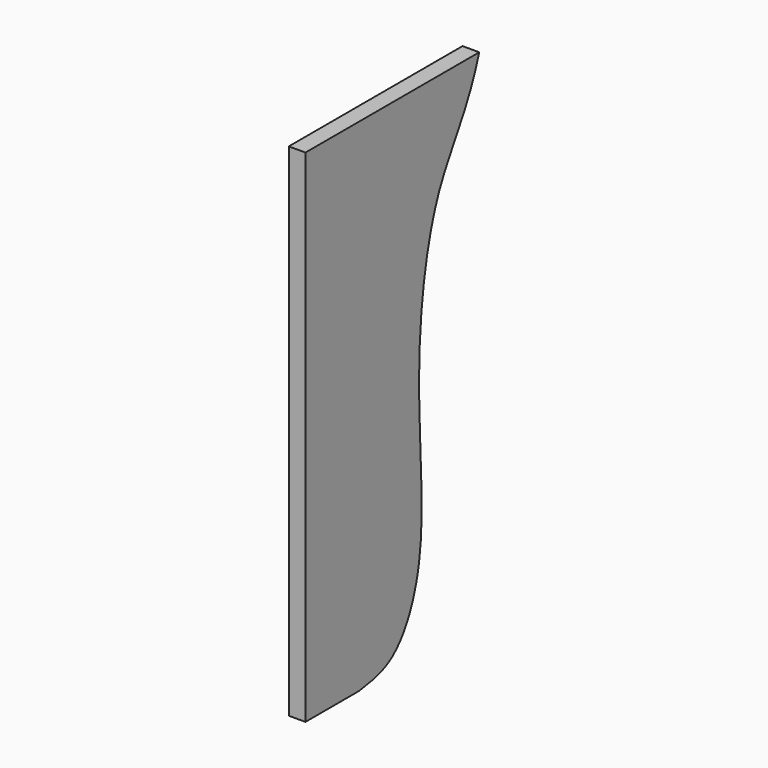
from build123d import *

# Parameters (mm, degrees)
F0_W     = 82.55
F0_H     = 190.5
F1_DEPTH = 6.35
F2_W     = 22.225
F2_H     = 5.08
F2_W_2   = 19.05
F2_H_2   = 26.4446459055
F2_H_3   = 61.5272244272
F2_H_4   = 58.6440721527
F3_DEPTH = 12.7


# Not quite as in the source:
# - a feature names something its author has since deleted; it is built from what else it names


with BuildPart() as f1:
    # F0 (on Right) → F1 (new body)
    with BuildSketch(Plane.YZ):
        with Locations((-52.8816960618, -14.7416193426)):
            Rectangle(F0_W, F0_H)
    extrude(amount=F1_DEPTH)

    # F2 (on face) → F3 (cut)
    with BuildSketch(Plane.YZ.offset(6.35)):
        with BuildLine():
            add(Edge.make_bspline(
                [(-52.8816960618, -104.9116193426), (-46.7384052574, -100.1821825443), (-42.1059434018, -90.4449211167), (-40.1816960618, -78.4669734371)],
                knots=[0.1290930094, 0.1290930094, 0.1290930094, 0.1290930094, 0.3003556222, 0.3003556222, 0.3003556222, 0.3003556222], degree=3))
            Line((-52.8816960618, -104.9116193426), (-30.6566960618, -104.9116193426))
            Line((-30.6566960618, -104.9116193426), (-30.6566960618, -78.4669734371))
            Line((-30.6566960618, -78.4669734371), (-40.1816960618, -78.4669734371))
        make_face()
        with Locations((-41.7691960618, -107.4516193426)):
            Rectangle(F2_W, F2_H)
        with BuildLine():
            add(Edge.make_bspline(
                [(-68.7566960618, -109.9916193426), (-63.0013923205, -109.1961470607), (-57.5123383521, -108.4765376811), (-52.8816960618, -104.9116193426)],
                knots=[0, 0, 0, 0, 0.1290930094, 0.1290930094, 0.1290930094, 0.1290930094], degree=3))
            Line((-68.7566960618, -109.9916193426), (-52.8816960618, -109.9916193426))
            Line((-52.8816960618, -109.9916193426), (-52.8816960618, -104.9116193426))
        make_face()
        with Locations((-21.1316960618, -107.4516193426)):
            Rectangle(F2_W_2, F2_H)
        with Locations((-21.1316960618, -91.6892963898)):
            Rectangle(F2_W_2, F2_H_2)
        with Locations((-21.1316960618, -47.7033612235)):
            Rectangle(F2_W_2, F2_H_3)
        with BuildLine():
            add(Edge.make_bspline(
                [(-40.1816960618, -78.4669734371), (-37.3949778969, -61.1203653983), (-40.2882470853, -39.0743255012), (-40.1816960618, -16.9397490099)],
                knots=[0.3003556222, 0.3003556222, 0.3003556222, 0.3003556222, 0.5483802, 0.5483802, 0.5483802, 0.5483802], degree=3))
            Line((-40.1816960618, -78.4669734371), (-30.6566960618, -78.4669734371))
            Line((-30.6566960618, -78.4669734371), (-30.6566960618, -16.9397490099))
            Line((-30.6566960618, -16.9397490099), (-40.1816960618, -16.9397490099))
        make_face()
        with BuildLine():
            add(Edge.make_bspline(
                [(-40.1816960618, -16.9397490099), (-40.0769921004, 4.8111245801), (-37.0755702459, 26.6474918057), (-30.6566960618, 41.7043231428)],
                knots=[0.5483802, 0.5483802, 0.5483802, 0.5483802, 0.7921052716, 0.7921052716, 0.7921052716, 0.7921052716], degree=3))
            Line((-40.1816960618, -16.9397490099), (-30.6566960618, -16.9397490099))
            Line((-30.6566960618, -16.9397490099), (-30.6566960618, 41.7043231428))
        make_face()
        with Locations((-21.1316960618, 12.3822870664)):
            Rectangle(F2_W_2, F2_H_4)
        with BuildLine():
            add(Edge.make_bspline(
                [(-30.6566960618, 41.7043231428), (-25.1814690079, 54.5476299155), (-17.2197388458, 62.4582162191), (-11.6066960618, 80.5083806574)],
                knots=[0.7921052716, 0.7921052716, 0.7921052716, 0.7921052716, 1, 1, 1, 1], degree=3))
            Line((-30.6566960618, 41.7043231428), (-11.6066960618, 41.7043231428))
            Line((-11.6066960618, 41.7043231428), (-11.6066960618, 80.5083806574))
        make_face()
    extrude(amount=-F3_DEPTH, mode=Mode.SUBTRACT)


solid = f1.part
